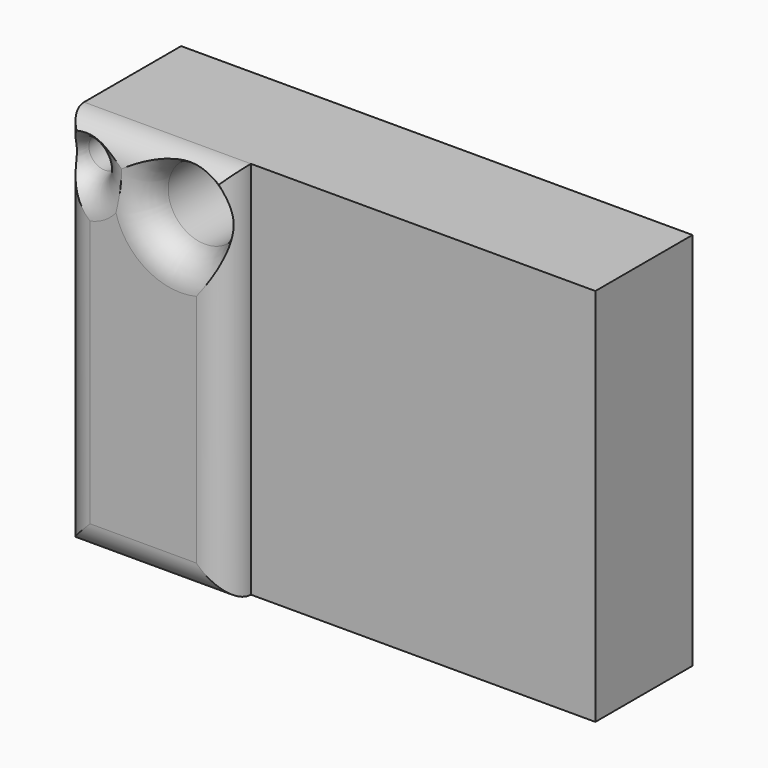
from build123d import *

# Parameters (mm, degrees)
F0_W        = 139.7
F0_H        = 317.5
F0_R        = 13.2493993782
F0_R_2      = 30.8467265461
F1_DEPTH    = 127
F2_T1_DEPTH = 266.7
F2_T3_DEPTH = 444.5
F3_DEPTH    = 288.29


# Not quite as in the source:
# - a fillet or chamfer that OpenCascade refuses, or shapes differently, is made with other operations: its cross-section is extruded or revolved along the edge and cut away or added


with BuildPart() as f1:
    # F0 (on Front) → F1 (new body)
    with BuildSketch(Plane.XZ):
        with Locations((18.042704469, 87.1669226885)):
            Rectangle(F0_W, F0_H)
        with Locations((-34.4466865063, 214.674949646)):
            Circle(F0_R, mode=Mode.SUBTRACT)
        with Locations((49.4750849903, 204.995855689)):
            Circle(F0_R_2, mode=Mode.SUBTRACT)
    extrude(amount=F1_DEPTH)

    # F2: fillet of radius 25.4 on 6 edges, made by hand

    # F2_s2 → F2_t1 (cut)
    with BuildSketch(Plane.YZ.offset(-115.307295531)):
        with BuildLine():
            ThreePointArc((-101.6, 245.9169226885), (-119.5605122421, 238.4774349306), (-127, 220.5169226885))
            Line((-127, 220.5169226885), (-127, 245.9169226885))
            Line((-127, 245.9169226885), (-101.6, 245.9169226885))
        make_face()
        with BuildLine():
            ThreePointArc((-101.6, -71.5830773115), (-119.5605122421, -64.1435895537), (-127, -46.1830773115))
            Line((-127, -46.1830773115), (-127, -71.5830773115))
            Line((-127, -71.5830773115), (-101.6, -71.5830773115))
        make_face()
    extrude(amount=F2_T1_DEPTH, mode=Mode.SUBTRACT)

    # F2_s4 → F2_t3 (cut)
    with BuildSketch(Plane.XY.offset(-135.0830773115)):
        with BuildLine():
            ThreePointArc((-51.807295531, -101.6), (-44.3678077732, -119.5605122421), (-26.407295531, -127))
            Line((-26.407295531, -127), (-51.807295531, -127))
            Line((-51.807295531, -127), (-51.807295531, -101.6))
        make_face()
        with BuildLine():
            ThreePointArc((87.892704469, -101.6), (80.4532167111, -119.5605122421), (62.492704469, -127))
            Line((62.492704469, -127), (87.892704469, -127))
            Line((87.892704469, -127), (87.892704469, -101.6))
        make_face()
    extrude(amount=F2_T3_DEPTH, mode=Mode.SUBTRACT)

    # F2_s5 → F2_t6 (revolve, cut)
    with BuildSketch(Plane.XY.offset(214.674949646)):
        with BuildLine():
            ThreePointArc((-21.197287128, -101.6), (-13.7577993702, -119.5605122421), (4.202712872, -127))
            Line((4.202712872, -127), (-21.197287128, -127))
            Line((-21.197287128, -127), (-21.197287128, -101.6))
        make_face()
    revolve(axis=Axis((-34.4466865063, -127, 214.674949646), (0, -1, 0)), mode=Mode.SUBTRACT)

    # F2_s7 → F2_t8 (revolve, cut)
    with BuildSketch(Plane.XY.offset(204.995855689)):
        with BuildLine():
            ThreePointArc((80.3218115364, -101.6), (87.7612992942, -119.5605122421), (105.7218115364, -127))
            Line((105.7218115364, -127), (80.3218115364, -127))
            Line((80.3218115364, -127), (80.3218115364, -101.6))
        make_face()
    revolve(axis=Axis((49.4750849903, -127, 204.995855689), (0, -1, 0)), mode=Mode.SUBTRACT)

    # F3 (add): a face of the model
    f3_faces = [f1.faces().sort_by_distance(p)[0] for p in [
        (87.892704469, -50.8, 87.1669226885),
    ]]
    extrude(f3_faces, amount=F3_DEPTH)


solid = f1.part
